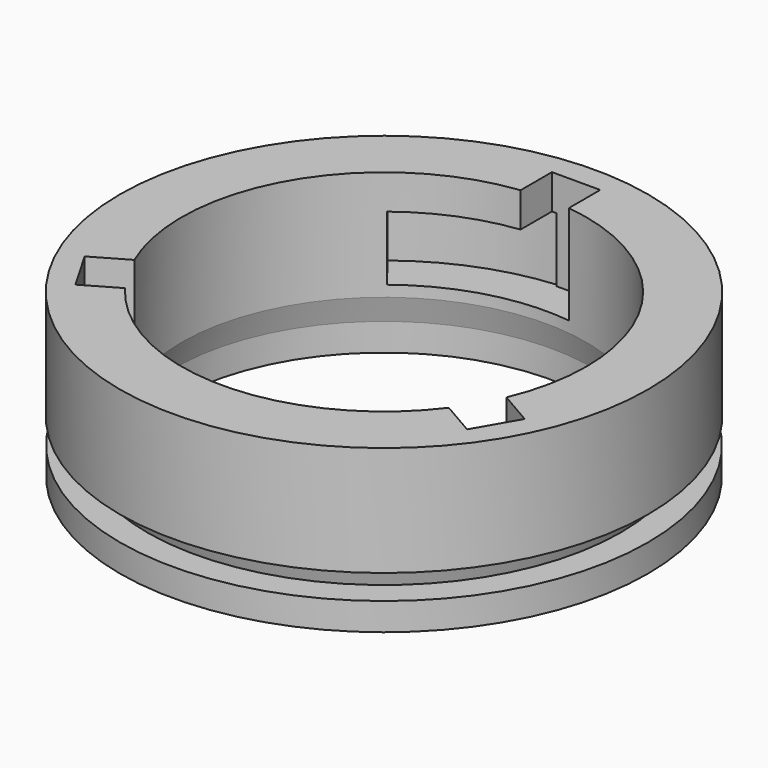
from build123d import *

# Parameters (mm, degrees)
F0_R      = 48
F0_R_2    = 42
F0_R_3    = 38
F1_DEPTH  = 5
F2_R      = 43.0776189128
F2_R_2    = 38
F3_DEPTH  = 4.5
F3_TAPER  = -15
F4_R      = 48.0278860385
F4_R_2    = 44.2833902788
F4_R_3    = 36.7942286341
F5_DEPTH  = 20
F7_DEPTH  = 18
F9_DEPTH  = 11.7
F10_R     = 1.9886860781
F11_DEPTH = 0.73


# Not quite as in the source:
# - a fillet or chamfer that OpenCascade refuses, or shapes differently, is made with other operations: its cross-section is extruded or revolved along the edge and cut away or added


with BuildPart() as f1:
    # F0 (on Top) → F1 (new body)
    with BuildSketch(Plane.XY):
        Circle(F0_R)
        Circle(F0_R_2, mode=Mode.SUBTRACT)
        Circle(F0_R_2)
        Circle(F0_R_3, mode=Mode.SUBTRACT)
    extrude(amount=F1_DEPTH)

    # F2 (on face) → F3 (join)
    with BuildSketch(Plane.XY.offset(5)):
        Circle(F2_R)
        Circle(F2_R_2, mode=Mode.SUBTRACT)
    extrude(amount=F3_DEPTH, taper=F3_TAPER)

    # F4 (on face) → F5 (join)
    with BuildSketch(Plane.XY.offset(9.5)):
        Circle(F4_R)
        Circle(F4_R_2, mode=Mode.SUBTRACT)
        Circle(F4_R_2)
        Circle(F4_R_3, mode=Mode.SUBTRACT)
    extrude(amount=F5_DEPTH)

    # F6 (on face) → F7 (cut)
    with BuildSketch(Plane.XY.offset(29.5)):
        Polygon((4.3897340074, 43.6625890434), (0, 43.6625890434), (-4.3897340074, 43.6625890434), (-4.3897340074, 34.0553857386), (0, 34.0553857386), (4.3897340074, 34.0553857386), align=None)
        Polygon((-35.6180443029, -25.632915688), (-27.2979621816, -20.8293140356), (-29.4928291853, -17.0276928693), (-31.687696189, -13.226071703), (-40.0077783103, -18.0296733554), (-37.8129113066, -21.8312945217), align=None)
        Polygon((40.0077783103, -18.0296733554), (31.687696189, -13.226071703), (29.4928291853, -17.0276928693), (27.2979621816, -20.8293140356), (35.6180443029, -25.632915688), (37.8129113066, -21.8312945217), align=None)
    extrude(amount=-F7_DEPTH, mode=Mode.SUBTRACT)

    # F8 (on face) → F9 (cut)
    with BuildSketch(Plane.XY.offset(11.5)):
        with BuildLine():
            ThreePointArc((-22.6687016251, 28.98180856), (-14.0459580236, 34.0077391776), (-4.3897340074, 36.5314316188))
            Line((-4.3897340074, 36.5314316188), (-4.3897340074, 43.6625890434))
            Line((-4.3897340074, 43.6625890434), (-3.592736461, 43.6625890434))
            Line((-3.592736461, 43.6625890434), (-3.592736461, 44.0917754576))
            ThreePointArc((-3.592736461, 44.0917754576), (-16.0835403712, 41.210582954), (-27.2238685762, 34.869089435))
            Line((-27.2238685762, 34.869089435), (-22.6687016251, 28.98180856))
        make_face()
        with BuildLine():
            ThreePointArc((36.4333332731, 5.1407671981), (36.7038939019, 2.5767097647), (36.7942286341, 0))
            ThreePointArc((36.7942286341, 0), (35.9635026363, -7.7744285261), (33.5088362695, -15.1978009146))
            Line((33.5088362695, -15.1978009146), (39.9809658747, -18.9344866844))
            ThreePointArc((39.9809658747, -18.9344866844), (43.7311819285, -6.6765369327), (43.8094515456, 6.1420170588))
            Line((43.8094515456, 6.1420170588), (36.4333332731, 5.1407671981))
        make_face()
        with BuildLine():
            Line((-16.5855829694, -41.0111064938), (-13.764631648, -34.1225757581))
            ThreePointArc((-13.764631648, -34.1225757581), (-22.7450346913, -28.9219407659), (-29.9160998084, -21.4206030033))
            Line((-29.9160998084, -21.4206030033), (-36.3882294137, -25.1572887731))
            ThreePointArc((-36.3882294137, -25.1572887731), (-27.6476415573, -34.5340460213), (-16.5855829694, -41.0111064938))
        make_face()
    extrude(amount=F9_DEPTH, mode=Mode.SUBTRACT)

    # F10 (on face) → F11 (join)
    with BuildSketch(Plane(origin=(0, 0, 23.2), x_dir=(1, 0, 0), z_dir=(0, 0, -1))):
        with Locations((-30.6445658207, 26.5157744288)):
            Circle(F10_R)
        with Locations((38.2856171667, 13.2810852742)):
            Circle(F10_R)
        with Locations((-7.6410513461, -39.7968597031)):
            Circle(F10_R)
    extrude(amount=F11_DEPTH)

    # F12: fillet of radius 1.6899494937 on 3 edges, made by hand

    # F12_s1 → F12_t2 (revolve, cut)
    with BuildSketch(Plane.XZ.offset(26.5157744288)):
        with BuildLine():
            ThreePointArc((-28.6558797426, 23.2), (-29.2613300231, 22.6635879979), (-30.0467162753, 22.47))
            Line((-30.0467162753, 22.47), (-28.6558797426, 22.47))
            Line((-28.6558797426, 22.47), (-28.6558797426, 23.2))
        make_face()
    revolve(axis=Axis((-30.6445658207, -26.5157744288, 22.47), (0, 0, -1)), mode=Mode.SUBTRACT)

    # F12_s3 → F12_t4 (revolve, cut)
    with BuildSketch(Plane.XZ.offset(13.2810852742)):
        with BuildLine():
            ThreePointArc((40.2743032449, 23.2), (39.6688529644, 22.6635879979), (38.8834667121, 22.47))
            Line((38.8834667121, 22.47), (40.2743032449, 22.47))
            Line((40.2743032449, 22.47), (40.2743032449, 23.2))
        make_face()
    revolve(axis=Axis((38.2856171667, -13.2810852742, 22.47), (0, 0, -1)), mode=Mode.SUBTRACT)

    # F12_s5 → F12_t6 (revolve, cut)
    with BuildSketch(Plane.XZ.offset(-39.7968597031)):
        with BuildLine():
            ThreePointArc((-5.6523652679, 23.2), (-6.2578155484, 22.6635879979), (-7.0432018006, 22.47))
            Line((-7.0432018006, 22.47), (-5.6523652679, 22.47))
            Line((-5.6523652679, 22.47), (-5.6523652679, 23.2))
        make_face()
    revolve(axis=Axis((-7.6410513461, 39.7968597031, 22.47), (0, 0, -1)), mode=Mode.SUBTRACT)


solid = f1.part
